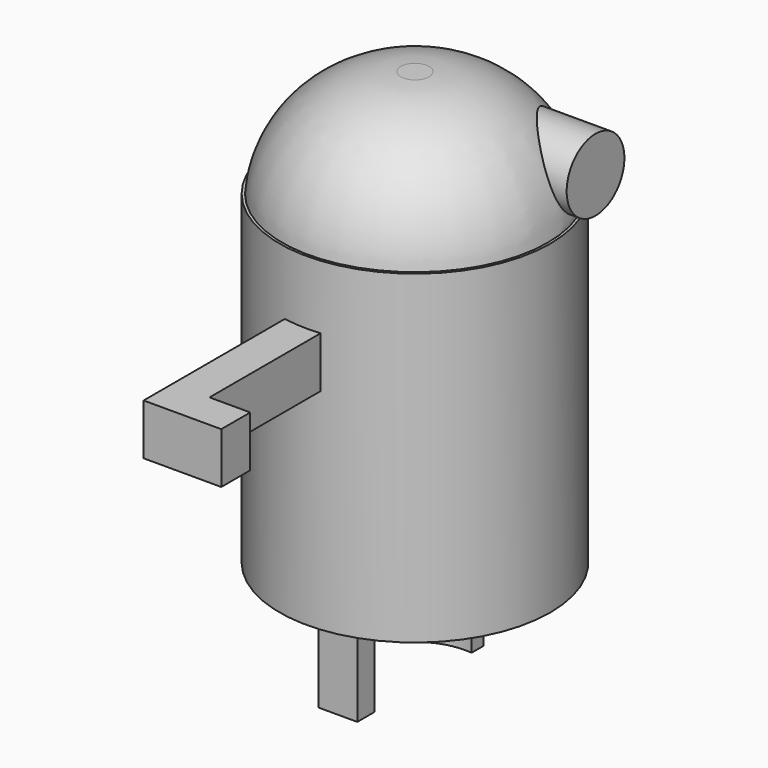
from build123d import *

# Parameters (mm, degrees)
F0_R      = 27.8562682198
F1_DEPTH  = 66.802
F2_R      = 27.3136197641
F3_DEPTH  = 22.098
F5_R      = 23.8036961542
F6_DEPTH  = 6.096
F9_DEPTH  = 15.24
F11_DEPTH = 14.986
F12_R     = 7.4259610206
F13_DEPTH = 28.194
F14_W     = 7.5996846426
F14_H     = 10.4752443731
F15_DEPTH = 63.754
F16_W     = 7.4501263418
F16_H     = 10.4752443731
F17_DEPTH = 8.382


# Not quite as in the source:
# - a fillet or chamfer that OpenCascade refuses, or shapes differently, is made with other operations: its cross-section is extruded or revolved along the edge and cut away or added


with BuildPart() as f1:
    # F0 (on Top) → F1 (new body)
    with BuildSketch(Plane.XY):
        Circle(F0_R)
    extrude(amount=F1_DEPTH)

    # F2 (on face) → F3 (join)
    with BuildSketch(Plane.XY.offset(66.802)):
        Circle(F2_R)
    extrude(amount=F3_DEPTH)

    # F4: fillet of radius 24.5284097937 on 1 edges, made by hand

    # F4_s1 → F4_t2 (revolve, cut)
    with BuildSketch(Plane.XZ):
        with BuildLine():
            ThreePointArc((27.3136197641, 66.802), (19.3684311501, 82.5547826432), (2.9059161596, 88.9))
            Line((2.9059161596, 88.9), (27.3136197641, 88.9))
            Line((27.3136197641, 88.9), (27.3136197641, 66.802))
        make_face()
    revolve(axis=Axis((0, 0, 88.9), (0, 0, 1)), mode=Mode.SUBTRACT)

    # F5 (on face) → F6 (join)
    with BuildSketch(Plane(origin=(0, 0, 0), x_dir=(1, 0, 0), z_dir=(0, 0, -1))):
        Circle(F5_R)
    extrude(amount=F6_DEPTH)

    # F7: fillet of radius 12.8774151417 on 1 edges, made by hand

    # F7_s1 → F7_t2 (revolve, cut)
    with BuildSketch(Plane.XZ):
        with BuildLine():
            ThreePointArc((23.8036961542, 0), (19.1215508115, -4.4692497), (12.8565399295, -6.096))
            Line((12.8565399295, -6.096), (23.8036961542, -6.096))
            Line((23.8036961542, -6.096), (23.8036961542, 0))
        make_face()
    revolve(axis=Axis((0, 0, -6.096), (0, 0, -1)), mode=Mode.SUBTRACT)

    # F12 (on Right) → F13 (join)
    with BuildSketch(Plane.YZ):
        with Locations((11.1912228167, 74.8514011502)):
            Circle(F12_R)
    extrude(amount=F13_DEPTH)

    # F14 (on Front) → F15 (join)
    with BuildSketch(Plane.XZ):
        with Locations((-1.0269851191, 48.4563689679)):
            Rectangle(F14_W, F14_H)
    extrude(amount=F15_DEPTH)

    # F16 (on face) → F17 (join)
    with BuildSketch(Plane.YZ.offset(2.7728572022)):
        with Locations((-60.0289368291, 48.4563689679)):
            Rectangle(F16_W, F16_H)
    extrude(amount=F17_DEPTH)


with BuildPart() as f9:
    # F8 (on face) → F9 (new body)
    with BuildSketch(Plane(origin=(0, 0, -6.096), x_dir=(1, 0, 0), z_dir=(0, 0, -1))):
        with BuildLine():
            ThreePointArc((-6.149337627, 11.2905387696), (-2.2848463598, 12.6518811278), (1.8117026193, 12.7282501774))
            Line((1.8117026193, 12.7282501774), (1.8117026193, 17.0915536582))
            Line((1.8117026193, 17.0915536582), (-6.149337627, 17.0915536582))
            Line((-6.149337627, 17.0915536582), (-6.149337627, 11.2905387696))
        make_face()
    extrude(amount=F9_DEPTH)


with BuildPart() as f11:
    # F10 (on face) → F11 (new body)
    with BuildSketch(Plane(origin=(0, 0, -6.096), x_dir=(1, 0, 0), z_dir=(0, 0, -1))):
        with BuildLine():
            Line((-6.505724193, -15.8313624561), (1.4219782315, -15.8313624561))
            Line((1.4219782315, -15.8313624561), (1.4219782315, -12.7776600701))
            ThreePointArc((1.4219782315, -12.7776600701), (-2.6784327348, -12.5744430113), (-6.505724193, -11.0890113032))
            Line((-6.505724193, -11.0890113032), (-6.505724193, -15.8313624561))
        make_face()
    extrude(amount=F11_DEPTH)


solid = Compound([f1.part, f9.part, f11.part])
